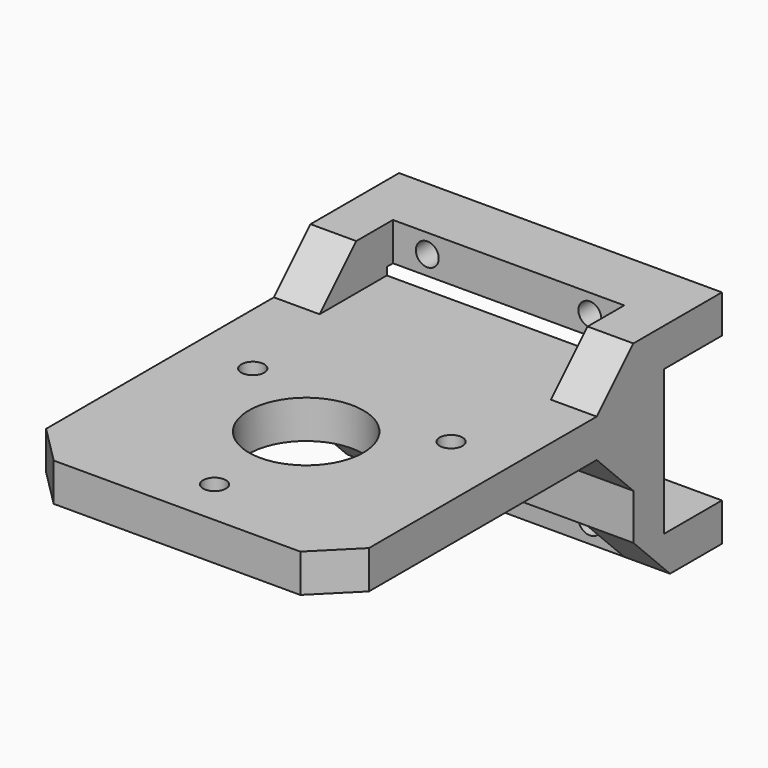
from build123d import *

# Parameters (mm, degrees)
F1_DEPTH  = 42.3
F3_W      = 30.3
F3_H      = 6
F4_DEPTH  = 6
F2_W      = 30.3
F2_H      = 6
F5_DEPTH  = 12
F6_SIZE   = 5.99999
F7_R      = 1.5
F8_DEPTH  = 8.501
F9_R      = 1.5
F10_DEPTH = 8.501
F11_R     = 1.5
F11_R_2   = 7.5
F12_DEPTH = 5
F13_SIZE  = 5


# Not quite as in the source:
# - a fillet or chamfer is up to 0.001 mm smaller than in the source, because OpenCascade refuses the exact size
# - a feature names something its author has since deleted; it is built from what else it names


with BuildPart() as f1:
    # F0 (on Right) → F1 (new body)
    with BuildSketch(Plane.YZ):
        Polygon((-9.5, 9.5), (0, 9.5), (0, 14.5), (-14.5, 14.5), (-20.5, 14.5), (-20.5, 8.5), (-62.8, 8.5), (-62.8, 3.5), (-20.5, 3.5), (-20.5, -2.5), (-14.5, -2.5), (-14.5, -14.5), (0, -14.5), (0, -9.5), (-9.5, -9.5), align=None)
    extrude(amount=F1_DEPTH)

    # F3 (on face) → F4 (cut)
    with BuildSketch(Plane.XZ.offset(14.5)):
        with Locations((21.15, -11.5)):
            Rectangle(F3_W, F3_H)
    extrude(amount=-F4_DEPTH, mode=Mode.SUBTRACT)

    # F2 (on face) → F5 (cut)
    with BuildSketch(Plane.XZ.offset(20.5)):
        with Locations((21.15, 11.5)):
            Rectangle(F2_W, F2_H)
    extrude(amount=-F5_DEPTH, mode=Mode.SUBTRACT)

    # F6 (size 6 in the source; OpenCascade refuses exactly that, so slightly less here)
    f6_edges = [f1.edges().sort_by_distance(p)[0] for p in [
        (3, -14.5, -14.5),
        (39.3, -14.5, -14.5),
        (3, -20.5, 14.5),
        (39.3, -20.5, 14.5),
        (21.15, -20.5, -2.5),
    ]]
    chamfer(f6_edges, length=F6_SIZE)

    # F7 (on face) → F8 (cut, through all)
    with BuildSketch(Plane.XZ.offset(8.5)):
        with Locations((10.5, 12)):
            Circle(F7_R)
        with Locations((31.8, 12)):
            Circle(F7_R)
    extrude(amount=-F8_DEPTH, mode=Mode.SUBTRACT)

    # F9 (on face) → F10 (cut, through all)
    with BuildSketch(Plane.XZ.offset(8.5)):
        with Locations((10.5, -12)):
            Circle(F9_R)
        with Locations((31.8, -12)):
            Circle(F9_R)
    extrude(amount=-F10_DEPTH, mode=Mode.SUBTRACT)

    # F11 (on face) → F12 (cut, through all)
    with BuildSketch(Plane.XY.offset(8.5)):
        with Locations((8.1596189432, -34.15)):
            Circle(F11_R)
        with Locations((21.15, -41.65)):
            Circle(F11_R_2)
        with Locations((34.1403810568, -34.15)):
            Circle(F11_R)
        with Locations((21.15, -56.65)):
            Circle(F11_R)
    extrude(amount=-F12_DEPTH, mode=Mode.SUBTRACT)

    # F13
    f13_edges = [f1.edges().sort_by_distance(p)[0] for p in [
        (42.3, -62.8, 6),
        (0, -62.8, 6),
    ]]
    chamfer(f13_edges, length=F13_SIZE)


solid = f1.part
